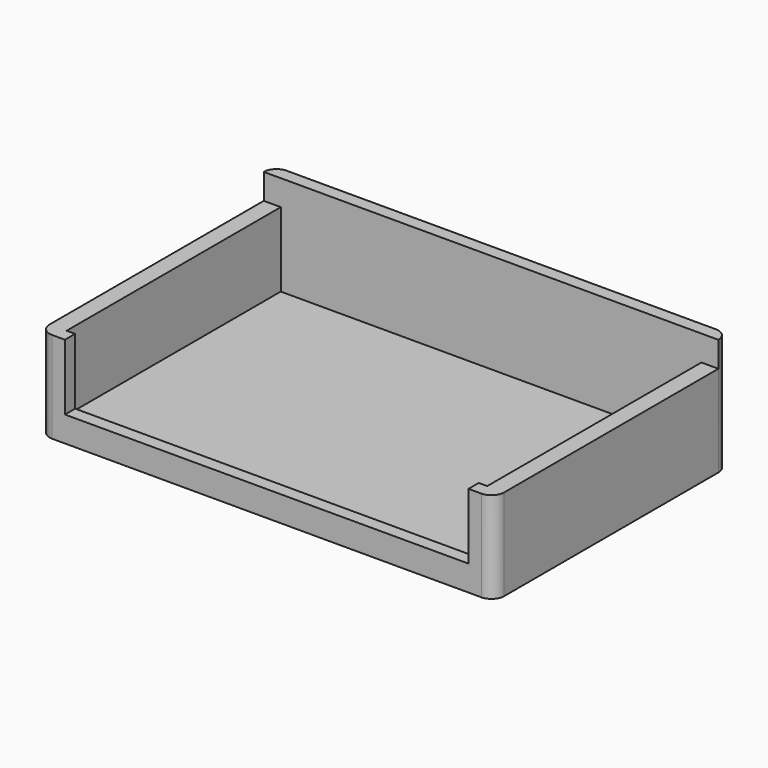
from build123d import *

# Parameters (mm, degrees)
F0_W     = 107
F0_H     = 6
F1_DEPTH = 69
F3_DEPTH = 15.5
F4_W     = 2
F4_H     = 63
F4_W_2   = 95
F5_DEPTH = 17.5
F6_DEPTH = 6
F7_R     = 2.99999


# Not quite as in the source:
# - a fillet or chamfer is up to 0.001 mm smaller than in the source, because OpenCascade refuses the exact size


with BuildPart() as f1:
    # F0 (on Front) → F1 (new body)
    with BuildSketch(Plane.XZ):
        with Locations((0, 3)):
            Rectangle(F0_W, F0_H)
    extrude(amount=F1_DEPTH)

    # F2 (on face) → F3 (join)
    with BuildSketch(Plane.XY.offset(6)):
        Polygon((53.5, -3), (53.5, 0), (47.5, 0), (-47.5, 0), (-53.5, 0), (-53.5, -3), (-53.5, -69), (-47.5, -69), (-47.5, -3), (47.5, -3), (47.5, -69), (53.5, -69), align=None)
    extrude(amount=F3_DEPTH)

    # F4 (on face) → F5 (cut)
    with BuildSketch(Plane.XY.offset(21.5)):
        with Locations((-48.5, -34.5)):
            Rectangle(F4_W, F4_H)
        with Locations((0, -34.5)):
            Rectangle(F4_W_2, F4_H)
        with Locations((48.5, -34.5)):
            Rectangle(F4_W, F4_H)
    extrude(amount=-F5_DEPTH, mode=Mode.SUBTRACT)

    # F4 (on face) → F6 (join)
    with BuildSketch(Plane.XY.offset(21.5)):
        Polygon((-53.5, -3), (-49.5, -3), (-47.5, -3), (47.5, -3), (49.5, -3), (53.5, -3), (53.5, 0), (-53.5, 0), align=None)
    extrude(amount=F6_DEPTH)

    # F7 (radius 3 in the source; OpenCascade refuses exactly that, so slightly less here)
    f7_edges = [f1.edges().sort_by_distance(p)[0] for p in [
        (-53.5, -69, 10.75),
        (53.5, -69, 10.75),
        (53.5, 0, 13.75),
        (-53.5, 0, 13.75),
    ]]
    fillet(f7_edges, radius=F7_R)


solid = f1.part
